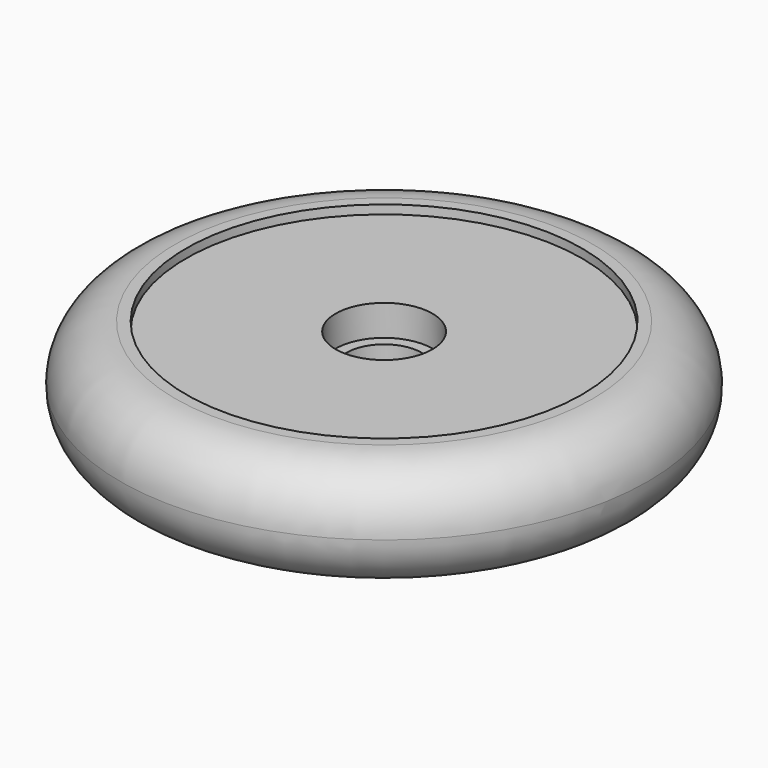
from build123d import *

# Parameters (mm, degrees)
F0_R      = 60
F1_DEPTH  = 25
F2_R      = 11
F4_DEPTH  = 9
F3_R      = 45
F3_R_2    = 11
F5_DEPTH  = 0.01
F6_DEPTH  = 2
F7_R      = 11
F9_DEPTH  = 9
F8_R      = 45
F10_DEPTH = 2
F11_R     = 12.5
F12_R     = 12.49999
F13_R     = 8.5
F14_DEPTH = 25


# Not quite as in the source:
# - a fillet or chamfer is up to 0.001 mm smaller than in the source, because OpenCascade refuses the exact size


with BuildPart() as f1:
    # F0 (on Top) → F1 (new body)
    with BuildSketch(Plane.XY):
        Circle(F0_R)
    extrude(amount=F1_DEPTH)

    # F2 (on face) → F4 (cut)
    with BuildSketch(Plane.XY.offset(25)):
        Circle(F2_R)
    extrude(amount=-F4_DEPTH, mode=Mode.SUBTRACT)

    # F3 (on face) → F5 (cut)
    with BuildSketch(Plane.XY.offset(25)):
        Circle(F3_R)
        Circle(F3_R_2, mode=Mode.SUBTRACT)
    extrude(amount=-F5_DEPTH, mode=Mode.SUBTRACT)

    # F3 (on face) → F6 (cut)
    with BuildSketch(Plane.XY.offset(25)):
        Circle(F3_R)
    extrude(amount=-F6_DEPTH, mode=Mode.SUBTRACT)

    # F7 (on face) → F9 (cut)
    with BuildSketch(Plane(origin=(0, 0, 0), x_dir=(1, 0, 0), z_dir=(0, 0, -1))):
        Circle(F7_R)
    extrude(amount=-F9_DEPTH, mode=Mode.SUBTRACT)

    # F8 (on face) → F10 (cut)
    with BuildSketch(Plane(origin=(0, 0, 0), x_dir=(1, 0, 0), z_dir=(0, 0, -1))):
        Circle(F8_R)
    extrude(amount=-F10_DEPTH, mode=Mode.SUBTRACT)

    # F11
    f11_edges = [f1.edges().sort_by_distance(p)[0] for p in [
        (-60, 0, 25),
    ]]
    fillet(f11_edges, radius=F11_R)

    # F12 (radius 12.5 in the source; OpenCascade refuses exactly that, so slightly less here)
    f12_edges = [f1.edges().sort_by_distance(p)[0] for p in [
        (-60, 0, 0),
    ]]
    fillet(f12_edges, radius=F12_R)

    # F13 (on face) → F14 (cut)
    with BuildSketch(Plane.XY.offset(16)):
        Circle(F13_R)
    extrude(amount=-F14_DEPTH, mode=Mode.SUBTRACT)


solid = f1.part
